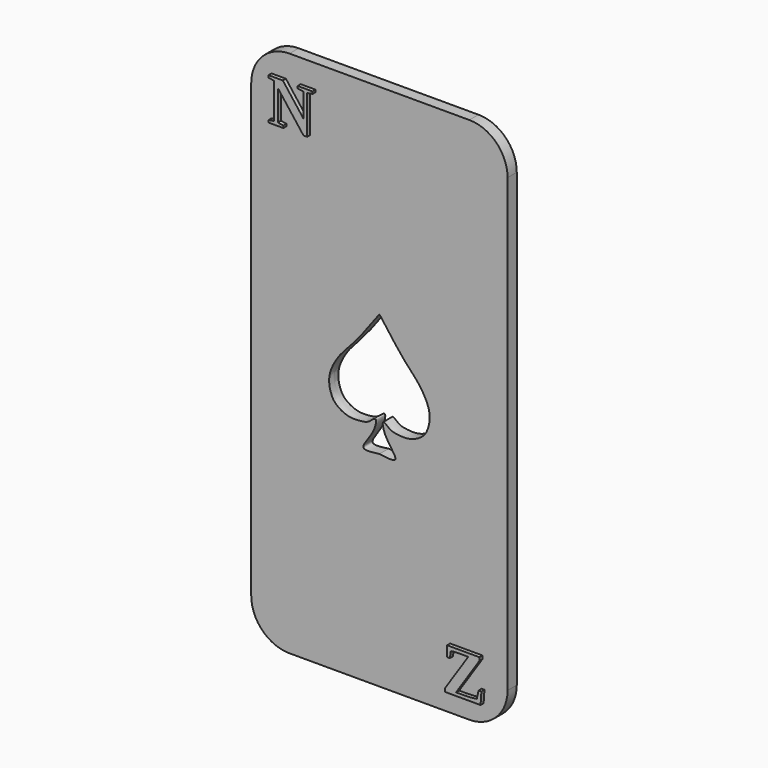
from build123d import *

# Parameters (mm, degrees)
F3_DEPTH     = 3
F4_DEPTH     = 12.5
F1_TEXT_SIZE = 16.6666666667
F5_DEPTH     = 4


# Not quite as in the source:
# - Text() gives the source's letters only with a copy of the font that has no kerning and outlines rounded to 1/6400 em; it was checked with that copy


with BuildPart() as f3:
    # F0 (on Front) → F3 (new body)
    with BuildSketch(Plane.XZ):
        with BuildLine():
            Line((23.5, 69), (-23.5, 69))
            ThreePointArc((-23.5, 69), (-30.5710678119, 66.0710678119), (-33.5, 59))
            Line((-33.5, 59), (-33.5, -59))
            ThreePointArc((-33.5, -59), (-30.5710678119, -66.0710678119), (-23.5, -69))
            Line((-23.5, -69), (23.5, -69))
            ThreePointArc((23.5, -69), (30.5710678119, -66.0710678119), (33.5, -59))
            Line((33.5, -59), (33.5, 59))
            ThreePointArc((33.5, 59), (30.5710678119, 66.0710678119), (23.5, 69))
        make_face()
    extrude(amount=F3_DEPTH)

    # F2 (on face) → F4 (cut, symmetric)
    with BuildSketch(Plane.XZ):
        with BuildLine():
            add(Edge.make_bspline(
                [(0, 16.667176038), (1.177592493, 15.058970665), (3.5138998516, 11.8683405705), (7.1548524343, 7.3142245777), (10.225785144, 4.2865675256), (12.2068576569, 1.0865621384), (13.1600146484, -1.5018160378), (13.1834658394, -3.9455250075), (12.5831356537, -5.840322962), (12.0199309955, -7.0692751506), (10.8235859299, -8.2300082719), (8.9580695287, -9.2813326959), (6.9005430467, -9.6730251767), (5.149922493, -9.5460174641), (4.5682527826, -9.4329691563), (3.6914891988, -9.3393939554), (2.5252599715, -8.9028494644), (0.4939053095, -6.8296584916), (1.1959875101, -11.2373780454), (6.076916012, -16.3284608774), (1.9493952073, -15.7534121812), (0, -15.4818212613)],
                knots=[0, 0, 0, 0, 0.0808440511, 0.1603921158, 0.2290636978, 0.2923055495, 0.3467263551, 0.3977534922, 0.4437608307, 0.4815229337, 0.523334574, 0.5714598493, 0.6200011904, 0.6627400882, 0.6878527305, 0.717281522, 0.7563945049, 0.7996537867, 0.8576775887, 0.9327822585, 1, 1, 1, 1], degree=3))
            add(Edge.make_bspline(
                [(0, 16.667176038), (-1.177592493, 15.058970665), (-3.5138998516, 11.8683405705), (-7.1548524343, 7.3142245777), (-10.225785144, 4.2865675256), (-12.2068576569, 1.0865621384), (-13.1600146484, -1.5018160378), (-13.1834658394, -3.9455250075), (-12.5831356537, -5.840322962), (-12.0199309955, -7.0692751506), (-10.8235859299, -8.2300082719), (-8.9580695287, -9.2813326959), (-6.9005430467, -9.6730251767), (-5.149922493, -9.5460174641), (-4.5682527826, -9.4329691563), (-3.6914891988, -9.3393939554), (-2.5252599715, -8.9028494644), (-0.4939053095, -6.8296584916), (-1.1959875101, -11.2373780454), (-6.076916012, -16.3284608774), (-1.9493952073, -15.7534121812), (0, -15.4818212613)],
                knots=[0, 0, 0, 0, 0.0808440511, 0.1603921158, 0.2290636978, 0.2923055495, 0.3467263551, 0.3977534922, 0.4437608307, 0.4815229337, 0.523334574, 0.5714598493, 0.6200011904, 0.6627400882, 0.6878527305, 0.717281522, 0.7563945049, 0.7996537867, 0.8576775887, 0.9327822585, 1, 1, 1, 1], degree=3))
        make_face()
    extrude(amount=F4_DEPTH, both=True, mode=Mode.SUBTRACT)

    # F1 (on face) → F5 (join)
    with BuildSketch(Plane.XZ):
        with Locations((-28.5, 52)):
            Text('N', F1_TEXT_SIZE, font='Tinos', font_style=FontStyle.BOLD, text_align=(TextAlign.LEFT, TextAlign.BOTTOM))
        with Locations((17.1875, -64)):
            Text('Z', F1_TEXT_SIZE, font='Tinos', font_style=FontStyle.BOLD, text_align=(TextAlign.LEFT, TextAlign.BOTTOM))
    extrude(amount=F5_DEPTH)


solid = f3.part
